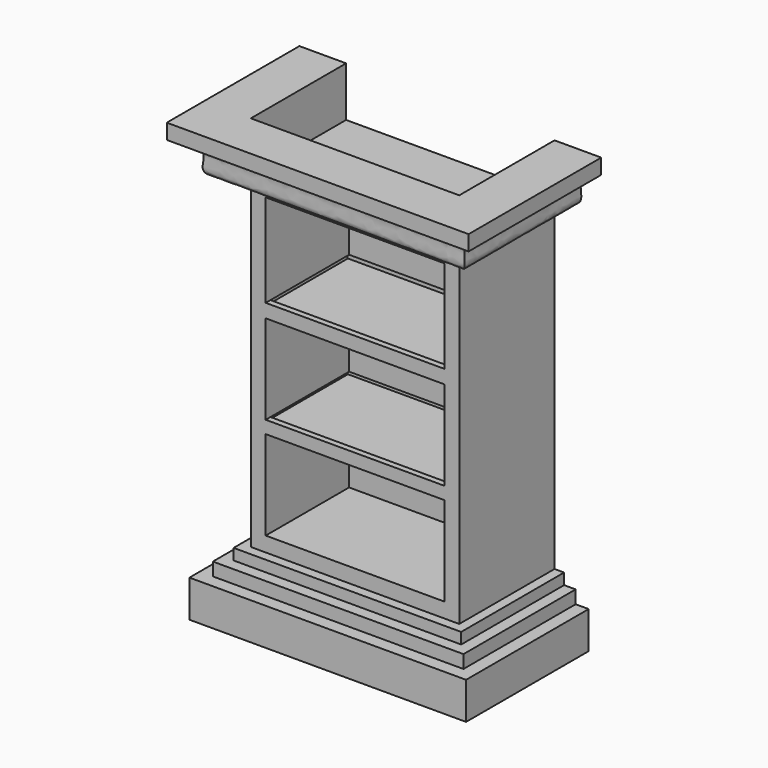
from build123d import *

# Parameters (mm, degrees)
F0_W      = 88.9
F0_H      = 139.7
F1_DEPTH  = 50.8
F2_T      = -6.35
F9_W      = 76.2
F9_H      = 5.8078249037
F9_H_2    = 5.3777060688
F10_DEPTH = 44.45
F11_T     = -2.54


# Not quite as in the source:
# - a shell that OpenCascade refuses in one call is made with other operations: the cavity is built on its own and cut out


with BuildPart() as f1:
    # F0 (on Front) → F1 (new body)
    with BuildSketch(Plane.XZ):
        with Locations((44.45, 69.85)):
            Rectangle(F0_W, F0_H)
    extrude(amount=F1_DEPTH)

    # F2
    f2_openings = [f1.faces().sort_by_distance(p)[0] for p in [
        (44.45, -50.8, 69.85),
    ]]
    offset(amount=F2_T, openings=f2_openings)

    # F9 (on face) → F10 (join)
    with BuildSketch(Plane.XZ.offset(6.35)):
        with Locations((44.45, 90.8316185206)):
            Rectangle(F9_W, F9_H)
        with Locations((44.45, 47.1388530344)):
            Rectangle(F9_W, F9_H_2)
    extrude(amount=F10_DEPTH)

    # F11: a shell. OpenCascade refuses it in one call, so the cavity is built on its own and cut out:
    # the body offset inwards by the wall thickness, plus a prism from it out through each open face.
    f11_core = offset(f1.part, amount=F11_T, kind=Kind.INTERSECTION, mode=Mode.PRIVATE)
    f11_exits = [f11_core.faces().sort_by_distance(p)[0] for p in [
        (44.45, -26.035, 91.195531),
        (44.45, -26.035, 47.287706),
    ]]
    add(f11_core, mode=Mode.SUBTRACT)
    extrude(f11_exits, amount=-F11_T, mode=Mode.SUBTRACT)


with BuildPart() as f5:
    # F5: sweep along a path in F3
    with BuildLine(Plane.XY.offset(139.7)) as f5_path:
        Line((0, 0), (0, -50.8))
        Line((0, -50.8), (88.9, -50.8))
        Line((88.9, -50.8), (88.9, 0))
    # F4 (on face) → F5 (sweep)
    with BuildSketch(Plane(origin=(0, 0, 0), x_dir=(-1, 0, 0), z_dir=(0, 1, 0))):
        with BuildLine():
            Line((0, 160.9531491995), (0, 139.7))
            Line((0, 139.7), (7.1226162836, 139.7))
            add(Edge.make_bspline(
                [(19.9233293533, 154.4612050056), (15.1122931258, 154.7714925538), (9.8517459293, 149.9580939303), (12.2362864635, 142.8802470964), (10.3562465476, 140.1408824591), (7.1226162836, 139.7)],
                knots=[0, 0, 0, 0, 0.3951929402, 0.7060594336, 1, 1, 1, 1], degree=3))
            Line((19.9233293533, 154.4612050056), (19.9233293533, 160.9531491995))
            Line((19.9233293533, 160.9531491995), (0, 160.9531491995))
        make_face()
    sweep(path=f5_path.line, transition=Transition.RIGHT)


with BuildPart() as f8:
    # F8: sweep along a path in F6
    with BuildLine(Plane(origin=(0, 0, 0), x_dir=(1, 0, 0), z_dir=(0, 0, -1))) as f8_path:
        Line((88.9, 0), (88.9, 50.8))
        Line((88.9, 50.8), (0, 50.8))
        Line((0, 50.8), (0, 0))
    # F7 (on face) → F8 (sweep)
    with BuildSketch(Plane(origin=(0, 0, 0), x_dir=(-1, 0, 0), z_dir=(0, 1, 0))):
        Polygon((4.080534447, 0), (0, 0), (0, -26.1282473803), (14.5531892776, -26.1282473803), (14.5531892776, -14.4312130287), (14.5531892776, -10.3144859895), (9.0009085834, -10.3144859895), (9.0009085834, -4.7345655039), (4.080534447, -4.7345655039), align=None)
    sweep(path=f8_path.line, transition=Transition.RIGHT)


solid = Compound([f1.part, f5.part, f8.part])
